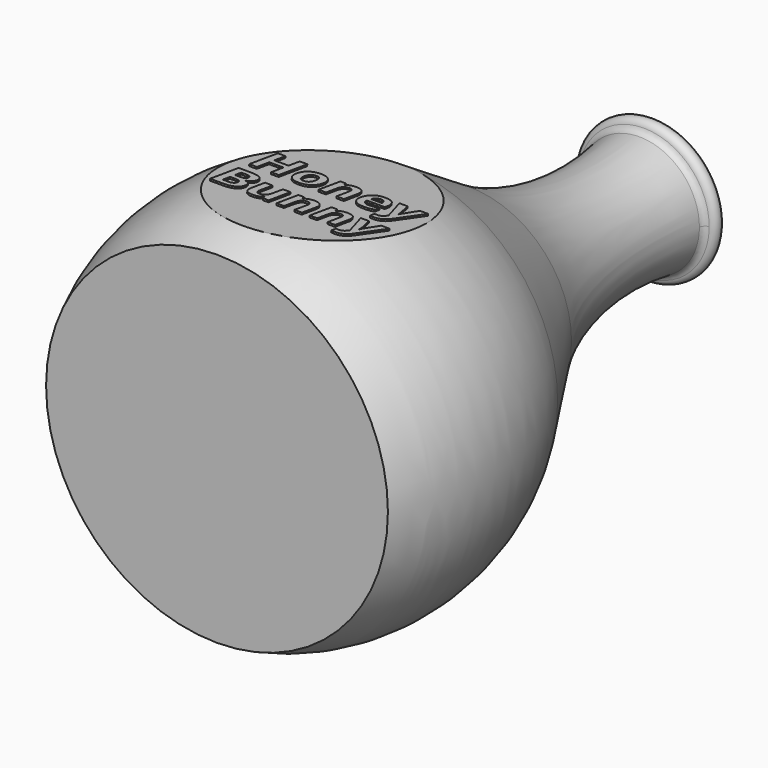
from build123d import *

# Parameters (mm, degrees)
F4_R         = 1.6
F6_DEPTH     = 25
F7_TEXT_SIZE = 11.8055555556
F9_DEPTH     = 0.4
F8_TEXT_SIZE = 11.8055555556
F10_DEPTH    = 0.4


# Not quite as in the source:
# - Text() gives the source's letters only with a copy of the font that has no kerning and outlines rounded to 1/6400 em; it was checked with that copy


with BuildPart() as f1:
    # F0 (on Top) → F1 (revolve)
    with BuildSketch(Plane.XY):
        with BuildLine():
            Line((0, 128), (0, 0))
            Line((0, 0), (40, 0))
            ThreePointArc((40, 0), (45.4058901196, 27.1900334558), (36.8625700808, 53.5629978328))
            Line((36.8625700808, 53.5629978328), (23.9930926245, 73.7279567282))
            ThreePointArc((23.9930926245, 73.7279567282), (13.9416746474, 99.9435141179), (15, 128))
            Line((15, 128), (0, 128))
        make_face()
    revolve(axis=Axis((0, 64, 0), (0, 1, 0)))

    # F2 (on Top) → F3 (revolve)
    with BuildSketch(Plane.XY):
        with BuildLine():
            Line((0, 124.8), (0, 128))
            Line((0, 128), (-15, 128))
            ThreePointArc((-15, 128), (-16.6, 126.4), (-15, 124.8))
            Line((-15, 124.8), (0, 124.8))
        make_face()
    revolve(axis=Axis((0, 126.4, 0), (0, 1, 0)))

    # F4
    f4_edges = [f1.edges().sort_by_distance(p)[0] for p in [
        (-14.297127, 124.8, 0),
    ]]
    fillet(f4_edges, radius=F4_R)

    # F5 (on Right) → F6 (cut, symmetric)
    with BuildSketch(Plane.YZ):
        Polygon((0, 44), (70, 34.1621415708), (70, 60), (0, 60), align=None)
    extrude(amount=F6_DEPTH, both=True, mode=Mode.SUBTRACT)

    # F7 (on face) → F9 (join)
    with BuildSketch(Plane(origin=(0, 6.064021828, 43.1477573106), x_dir=(1, 0, 0), z_dir=(0, 0.139173101, 0.9902680687))):
        with Locations((-18.8962673611, 25.8763835578)):
            Text('Honey', F7_TEXT_SIZE, font='Open Sans', font_style=FontStyle.BOLD, text_align=(TextAlign.LEFT, TextAlign.BOTTOM))
    extrude(amount=F9_DEPTH)

    # F8 (on face) → F10 (join)
    with BuildSketch(Plane(origin=(0, 6.064021828, 43.1477573106), x_dir=(1, 0, 0), z_dir=(0, 0.139173101, 0.9902680687))):
        with Locations((-18.9617513021, 14.3763835578)):
            Text('Bunny', F8_TEXT_SIZE, font='Open Sans', font_style=FontStyle.BOLD, text_align=(TextAlign.LEFT, TextAlign.BOTTOM))
    extrude(amount=F10_DEPTH)


solid = f1.part
